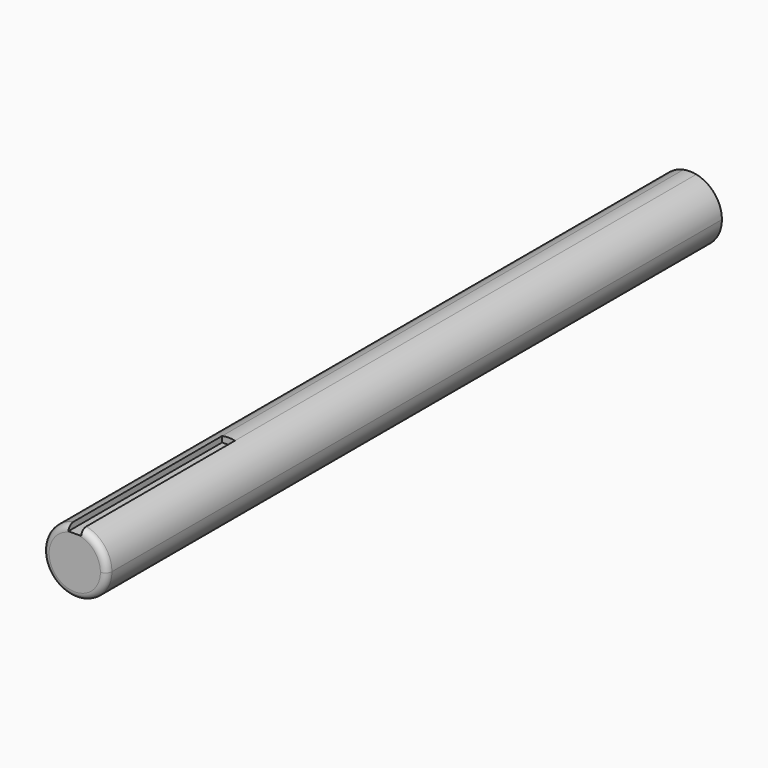
from build123d import *

# Parameters (mm, degrees)
F1_DEPTH = 600
F3_DEPTH = 150
F4_R     = 4.99999


# Not quite as in the source:
# - a fillet or chamfer is up to 0.001 mm smaller than in the source, because OpenCascade refuses the exact size


with BuildPart() as f1:
    # F0 (on Front) → F1 (new body)
    with BuildSketch(Plane.XZ):
        with BuildLine():
            ThreePointArc((-5, 24.4948974278), (-15.8113883008, -19.364916731), (25, 0))
            ThreePointArc((25, 0), (19.364916731, 15.8113883008), (5, 24.4948974278))
            Line((5, 24.4948974278), (5, 20))
            Line((5, 20), (0, 20))
            Line((0, 20), (-5, 20))
            Line((-5, 20), (-5, 24.4948974278))
        make_face()
        with BuildLine():
            Line((5, 20), (5, 24.4948974278))
            ThreePointArc((5, 24.4948974278), (0, 25), (-5, 24.4948974278))
            Line((-5, 24.4948974278), (-5, 20))
            Line((-5, 20), (0, 20))
            Line((0, 20), (5, 20))
        make_face()
    extrude(amount=F1_DEPTH)

    # F2 (on face) → F3 (cut)
    with BuildSketch(Plane.XZ.offset(600)):
        with BuildLine():
            Line((-5, 20), (0, 20))
            Line((0, 20), (5, 20))
            Line((5, 20), (5, 24.4948974278))
            ThreePointArc((5, 24.4948974278), (0, 25), (-5, 24.4948974278))
            Line((-5, 24.4948974278), (-5, 20))
        make_face()
    extrude(amount=-F3_DEPTH, mode=Mode.SUBTRACT)

    # F4 (radius 5 in the source; OpenCascade refuses exactly that, so slightly less here)
    f4_edges = [f1.edges().sort_by_distance(p)[0] for p in [
        (-15.811388, -600, -19.364917),
    ]]
    fillet(f4_edges, radius=F4_R)


solid = f1.part
